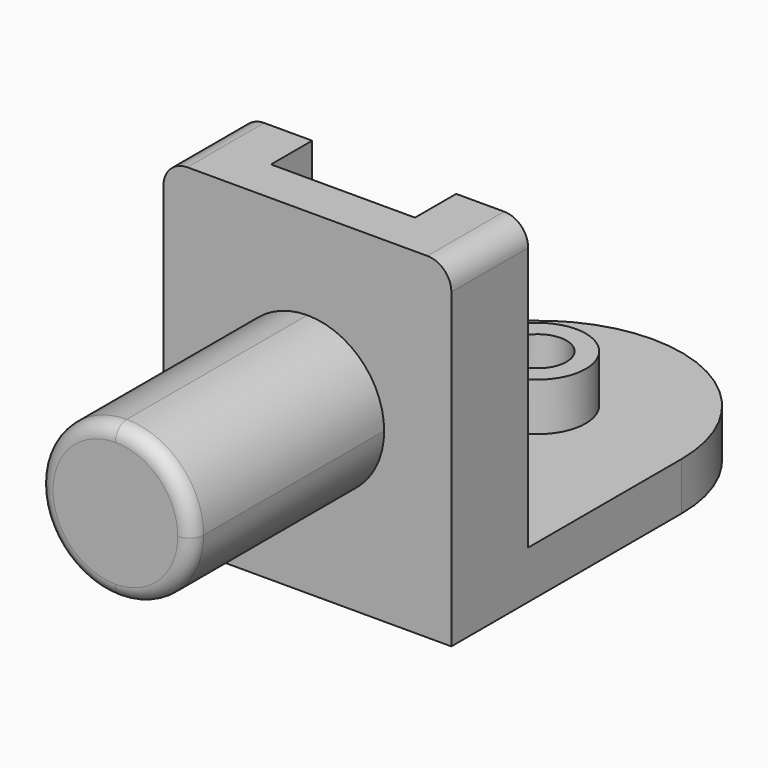
from build123d import *

# Parameters (mm, degrees)
F0_R      = 10
F1_DEPTH  = 10
F0_R_2    = 6
F2_DEPTH  = 20
F3_DEPTH  = 70
F5_DEPTH  = 60
F6_DEPTH  = 15
F8_R      = 5
F9_DEPTH  = 15
F10_R     = 5
F12_DEPTH = 50
F13_R     = 3


# Not quite as in the source:
# - a feature names something its author has since deleted; it is built from what else it names


with BuildPart() as f1:
    # F0 (on Top) → F1 (new body)
    with BuildSketch(Plane.XY):
        with BuildLine():
            Line((-35.661008209, 60), (-35.661008209, 20))
            Line((-35.661008209, 20), (24.338991791, 20))
            Line((24.338991791, 20), (24.338991791, 60))
            ThreePointArc((24.338991791, 60), (15.5521952266, 81.2132034356), (-5.661008209, 90))
            ThreePointArc((-5.661008209, 90), (-26.8742116446, 81.2132034356), (-35.661008209, 60))
        make_face()
        with Locations((-5.661008209, 60)):
            Circle(F0_R, mode=Mode.SUBTRACT)
    extrude(amount=F1_DEPTH)

    # F0 (on Top) → F3 (join)
    with BuildSketch(Plane.XY):
        Polygon((-35.661008209, 0), (-21.661008209, 0), (10.338991791, 0), (24.338991791, 0), (24.338991791, 20), (-35.661008209, 20), align=None)
    extrude(amount=F3_DEPTH)

    # F4 (on face) → F5 (cut)
    with BuildSketch(Plane(origin=(-35.661008209, 0, 0), x_dir=(0, -1, 0), z_dir=(-1, 0, 0))):
        Polygon((-9.2820323028, 70), (-20, 70), (-20, 30), align=None)
    extrude(amount=-F5_DEPTH, mode=Mode.SUBTRACT)

    # F4 (on face) → F6 (join)
    with BuildSketch(Plane(origin=(-35.661008209, 0, 0), x_dir=(0, -1, 0), z_dir=(-1, 0, 0))):
        Polygon((-9.2820323028, 70), (-20, 70), (-20, 30), align=None)
    extrude(amount=-F6_DEPTH)

    # F8
    f8_edges = [f1.edges().sort_by_distance(p)[0] for p in [
        (-35.661008, 10, 70),
    ]]
    fillet(f8_edges, radius=F8_R)

    # F7 (on face) → F9 (join)
    with BuildSketch(Plane.YZ.offset(24.338991791)):
        Polygon((20, 70), (9.2820323028, 70), (20, 30), align=None)
    extrude(amount=-F9_DEPTH)

    # F10
    f10_edges = [f1.edges().sort_by_distance(p)[0] for p in [
        (24.338992, 10, 70),
    ]]
    fillet(f10_edges, radius=F10_R)

    # F11 (on face) → F12 (join)
    with BuildSketch(Plane.XZ):
        with BuildLine():
            Line((-5.661008209, 35), (-5.661008209, 19))
            ThreePointArc((-5.661008209, 19), (5.65270029, 23.686291501), (10.338991791, 35))
            ThreePointArc((10.338991791, 35), (5.65270029, 46.313708499), (-5.661008209, 51))
            Line((-5.661008209, 51), (-5.661008209, 35))
        make_face()
        with BuildLine():
            ThreePointArc((-5.661008209, 51), (-21.661008209, 35), (-5.661008209, 19))
            Line((-5.661008209, 19), (-5.661008209, 35))
            Line((-5.661008209, 35), (-5.661008209, 51))
        make_face()
    extrude(amount=F12_DEPTH)

    # F13
    f13_edges = [f1.edges().sort_by_distance(p)[0] for p in [
        (-5.661008, -50, 19),
    ]]
    fillet(f13_edges, radius=F13_R)


with BuildPart() as f2:
    # F0 (on Top) → F2 (new body)
    with BuildSketch(Plane.XY):
        with Locations((-5.661008209, 60)):
            Circle(F0_R)
        with Locations((-5.661008209, 60)):
            Circle(F0_R_2, mode=Mode.SUBTRACT)
    extrude(amount=F2_DEPTH)


solid = Compound([f1.part, f2.part])
